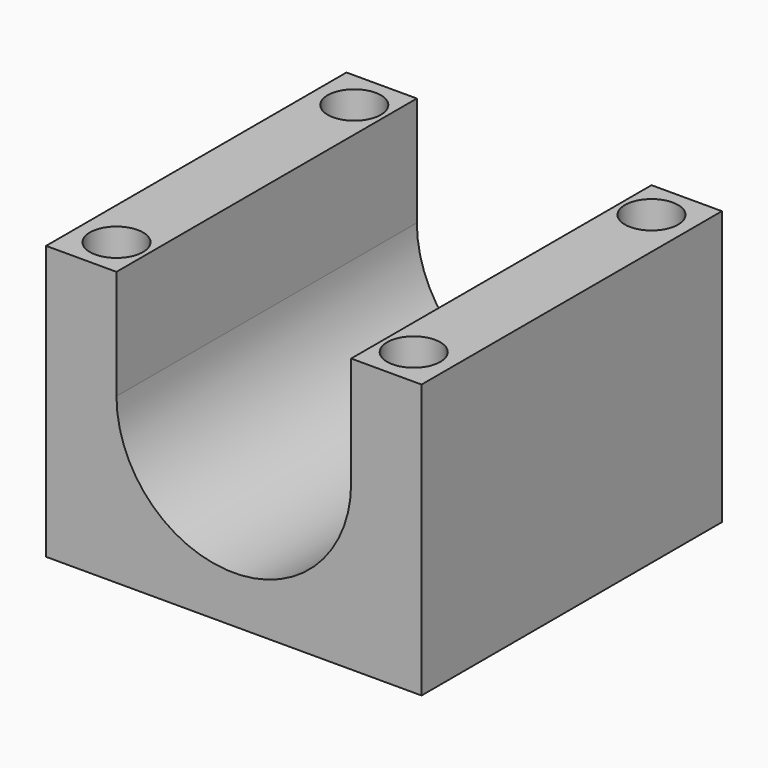
from build123d import *

# Parameters (mm, degrees)
F0_W            = 24
F0_H            = 24
F1_DEPTH        = 17.5
F3_DEPTH        = 25
F5_D            = 3.4
F5_COPIES_COUNT = 4


# Not quite as in the source:
# - a pattern or mirror of a feature is missing from the dataset's text; its kind, count and spacing are read off the source's solid


with BuildPart() as f1:
    # F0 (on Top) → F1 (new body)
    with BuildSketch(Plane.XY):
        Rectangle(F0_W, F0_H)
    extrude(amount=F1_DEPTH)

    # F2 (on face) → F3 (cut)
    with BuildSketch(Plane.XZ.offset(12)):
        with BuildLine():
            ThreePointArc((-7.5, 10.5), (0, 3), (7.5, 10.5))
            Line((7.5, 10.5), (-7.5, 10.5))
        make_face()
        with BuildLine():
            ThreePointArc((7.5, 10.5), (6.1824092402, 14.7459175671), (2.6925824036, 17.5))
            Line((2.6925824036, 17.5), (-2.6925824036, 17.5))
            ThreePointArc((-2.6925824036, 17.5), (-6.1824092402, 14.7459175671), (-7.5, 10.5))
            Line((-7.5, 10.5), (7.5, 10.5))
        make_face()
        with BuildLine():
            Line((7.5, 10.5), (7.5, 17.5))
            Line((7.5, 17.5), (2.6925824036, 17.5))
            ThreePointArc((2.6925824036, 17.5), (6.1824092402, 14.7459175671), (7.5, 10.5))
        make_face()
        with BuildLine():
            ThreePointArc((-7.5, 10.5), (-6.1824092402, 14.7459175671), (-2.6925824036, 17.5))
            Line((-2.6925824036, 17.5), (-7.5, 17.5))
            Line((-7.5, 17.5), (-7.5, 10.5))
        make_face()
    extrude(amount=-F3_DEPTH, mode=Mode.SUBTRACT)

    # F5 (through all)
    with Locations(Plane.XY.offset(17.5)):
        with Locations((-9.5, -9.5)):
            f5 = Hole(F5_D / 2)

    # F5_copies: F5 ×4 about axis
    f5_copies_axis = Axis((0, 0, 0), (0, 0, 1))
    for i in range(1, F5_COPIES_COUNT):
        add(f5.rotate(f5_copies_axis, i * 360 / F5_COPIES_COUNT), mode=Mode.SUBTRACT)


solid = f1.part
